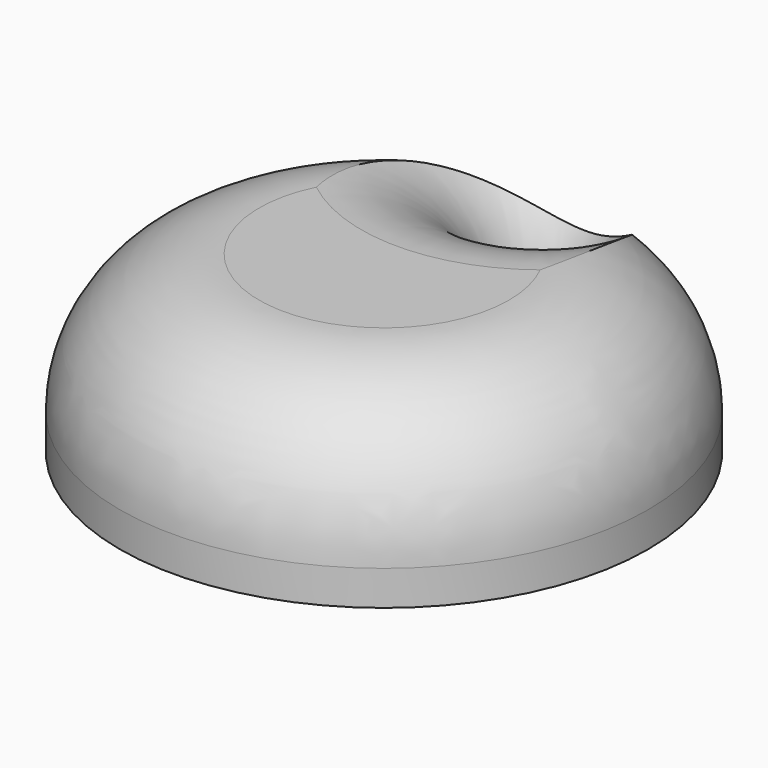
from build123d import *

# Parameters (mm, degrees)
F0_R     = 9.6376461191
F1_DEPTH = 6.35
F3_D     = 3.048


# Not quite as in the source:
# - a fillet or chamfer that OpenCascade refuses, or shapes differently, is made with other operations: its cross-section is extruded or revolved along the edge and cut away or added
# - a length typed as a fraction of an inch, garbled in the dataset ("3 / 203.2 mm" for 3/8 in), is restored


with BuildPart() as f1:
    # F0 (on Top) → F1 (new body)
    with BuildSketch(Plane.XY):
        Circle(F0_R)
    extrude(amount=F1_DEPTH)

    # F3 (through all)
    with Locations(Plane.XY.offset(6.35)):
        with Locations((0, 7.2102034464)):
            Hole(F3_D / 2)

    # F4: fillet of radius 5.08 on 2 edges, made by hand

    # F4_s1 → F4_t2 (revolve, cut)
    with BuildSketch(Plane.XZ):
        with BuildLine():
            ThreePointArc((9.6376461191, 1.27), (8.1497485675, 4.8621024484), (4.5576461191, 6.35))
            Line((4.5576461191, 6.35), (9.6376461191, 6.35))
            Line((9.6376461191, 6.35), (9.6376461191, 1.27))
        make_face()
    revolve(axis=Axis((0, 0, 6.35), (0, 0, 1)), mode=Mode.SUBTRACT)

    # F4_s3 → F4_t4 (revolve, cut)
    with BuildSketch(Plane.XZ.offset(-7.2102034464)):
        with BuildLine():
            ThreePointArc((6.604, 6.35), (3.0118975516, 4.8621024484), (1.524, 1.27))
            Line((1.524, 1.27), (1.524, 6.35))
            Line((1.524, 6.35), (6.604, 6.35))
        make_face()
    revolve(axis=Axis((0, 7.2102034464, 6.35), (0, 0, 1)), mode=Mode.SUBTRACT)


solid = f1.part
